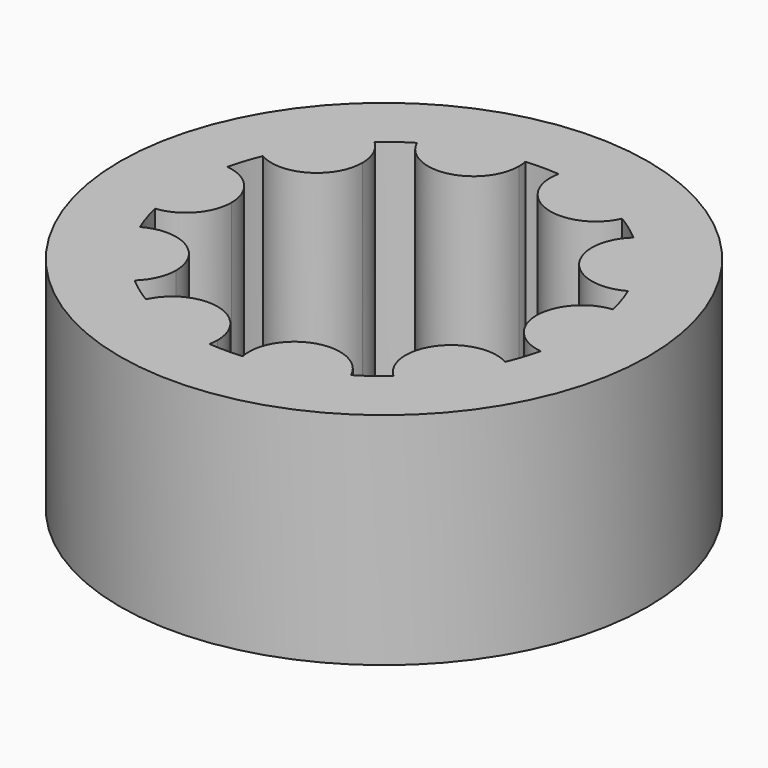
from build123d import *

# Parameters (mm, degrees)
F0_R     = 6
F1_DEPTH = 5


with BuildPart() as f1:
    # F0 (on Top) → F1 (new body)
    with BuildSketch(Plane.XY):
        with Locations((0.1191368553, 0.0803260972)):
            Circle(F0_R)
        with BuildLine():
            ThreePointArc((4.2675466454, 1.8240853161), (4.3988911787, 1.4709025719), (4.5002268275, 1.1079693501))
            ThreePointArc((4.5002268275, 1.1079693501), (5.3073148215, 0.8527258233), (5.6536368553, 0.0803260972))
            ThreePointArc((5.6536368553, 0.0803260972), (5.3073148215, -0.6920736289), (4.5002268275, -0.9473171557))
            ThreePointArc((4.5002268275, -0.9473171557), (4.3988911787, -1.3102503775), (4.2675466454, -1.6634331217))
            ThreePointArc((4.2675466454, -1.6634331217), (4.6528941109, -2.0427704321), (4.79421333, -2.5647075381))
            ThreePointArc((4.79421333, -2.5647075381), (4.1755248273, -3.5119620175), (3.059479548, -3.3261948332))
            ThreePointArc((3.059479548, -3.3261948332), (2.7641704906, -3.5602503775), (2.4503149228, -3.76877884))
            ThreePointArc((2.4503149228, -3.76877884), (2.5204661677, -3.9790445807), (2.54421333, -4.1994282261))
            ThreePointArc((2.54421333, -4.1994282261), (1.6124558319, -5.2288135905), (0.4956212985, -4.4038972987))
            ThreePointArc((0.4956212985, -4.4038972987), (0.1191368553, -4.4196739028), (-0.2573475879, -4.4038972987))
            ThreePointArc((-0.2573475879, -4.4038972987), (-1.5911177, -5.1832961922), (-2.2120412121, -3.76877884))
            ThreePointArc((-2.2120412121, -3.76877884), (-2.52589678, -3.5602503775), (-2.8212058374, -3.3261948332))
            ThreePointArc((-2.8212058374, -3.3261948332), (-4.3583677, -3.1727713816), (-4.0292729348, -1.6634331217))
            ThreePointArc((-4.0292729348, -1.6634331217), (-4.160617468, -1.3102503775), (-4.2619531169, -0.9473171557))
            ThreePointArc((-4.2619531169, -0.9473171557), (-5.4153631447, 0.0803260972), (-4.2619531169, 1.1079693501))
            ThreePointArc((-4.2619531169, 1.1079693501), (-4.160617468, 1.4709025719), (-4.0292729348, 1.8240853161))
            ThreePointArc((-4.0292729348, 1.8240853161), (-4.3583677, 3.333423576), (-2.8212058374, 3.4868470276))
            ThreePointArc((-2.8212058374, 3.4868470276), (-2.52589678, 3.7209025719), (-2.2120412121, 3.9294310345))
            ThreePointArc((-2.2120412121, 3.9294310345), (-1.5911177, 5.3439483866), (-0.2573475879, 4.5645494931))
            ThreePointArc((-0.2573475879, 4.5645494931), (0.1191368553, 4.5803260972), (0.4956212985, 4.5645494931))
            ThreePointArc((0.4956212985, 4.5645494931), (1.6124558319, 5.3894657849), (2.54421333, 4.3600804205))
            ThreePointArc((2.54421333, 4.3600804205), (2.5204661677, 4.1396967751), (2.4503149228, 3.9294310345))
            ThreePointArc((2.4503149228, 3.9294310345), (2.7641704906, 3.7209025719), (3.059479548, 3.4868470276))
            ThreePointArc((3.059479548, 3.4868470276), (4.1755248273, 3.6726142119), (4.79421333, 2.7253597325))
            ThreePointArc((4.79421333, 2.7253597325), (4.6528941109, 2.2034226265), (4.2675466454, 1.8240853161))
        make_face(mode=Mode.SUBTRACT)
        with BuildLine():
            ThreePointArc((4.5002268275, -0.9473171557), (4.5893105027, -0.4369239028), (4.6191368553, 0.0803260972))
            ThreePointArc((4.6191368553, 0.0803260972), (4.5893105027, 0.5975760972), (4.5002268275, 1.1079693501))
            ThreePointArc((4.5002268275, 1.1079693501), (3.5846368553, 0.0803260972), (4.5002268275, -0.9473171557))
        make_face()
        with BuildLine():
            ThreePointArc((4.5002268275, 1.1079693501), (4.5893105027, 0.5975760972), (4.6191368553, 0.0803260972))
            ThreePointArc((4.6191368553, 0.0803260972), (4.5893105027, -0.4369239028), (4.5002268275, -0.9473171557))
            ThreePointArc((4.5002268275, -0.9473171557), (5.3073148215, -0.6920736289), (5.6536368553, 0.0803260972))
            ThreePointArc((5.6536368553, 0.0803260972), (5.3073148215, 0.8527258233), (4.5002268275, 1.1079693501))
        make_face()
        with BuildLine():
            ThreePointArc((3.059479548, 3.4868470276), (2.9227852493, 2.117295889), (4.2675466454, 1.8240853161))
            ThreePointArc((4.2675466454, 1.8240853161), (3.75971333, 2.7253597325), (3.059479548, 3.4868470276))
        make_face()
        with BuildLine():
            ThreePointArc((3.059479548, 3.4868470276), (3.75971333, 2.7253597325), (4.2675466454, 1.8240853161))
            ThreePointArc((4.2675466454, 1.8240853161), (4.6528941109, 2.2034226265), (4.79421333, 2.7253597325))
            ThreePointArc((4.79421333, 2.7253597325), (4.1755248273, 3.6726142119), (3.059479548, 3.4868470276))
        make_face()
        with BuildLine():
            ThreePointArc((4.79421333, -2.5647075381), (4.6528941109, -2.0427704321), (4.2675466454, -1.6634331217))
            ThreePointArc((4.2675466454, -1.6634331217), (3.75971333, -2.5647075381), (3.059479548, -3.3261948332))
            ThreePointArc((3.059479548, -3.3261948332), (4.1755248273, -3.5119620175), (4.79421333, -2.5647075381))
        make_face()
        with BuildLine():
            ThreePointArc((3.059479548, -3.3261948332), (3.75971333, -2.5647075381), (4.2675466454, -1.6634331217))
            ThreePointArc((4.2675466454, -1.6634331217), (2.9227852493, -1.9566436946), (3.059479548, -3.3261948332))
        make_face()
        with BuildLine():
            ThreePointArc((0.4956212985, 4.5645494931), (1.1900352493, 3.3762124544), (2.4503149228, 3.9294310345))
            ThreePointArc((2.4503149228, 3.9294310345), (1.50971333, 4.3600804205), (0.4956212985, 4.5645494931))
        make_face()
        with BuildLine():
            ThreePointArc((0.4956212985, 4.5645494931), (1.50971333, 4.3600804205), (2.4503149228, 3.9294310345))
            ThreePointArc((2.4503149228, 3.9294310345), (2.5204661677, 4.1396967751), (2.54421333, 4.3600804205))
            ThreePointArc((2.54421333, 4.3600804205), (1.6124558319, 5.3894657849), (0.4956212985, 4.5645494931))
        make_face()
        with BuildLine():
            ThreePointArc((2.54421333, -4.1994282261), (2.5204661677, -3.9790445807), (2.4503149228, -3.76877884))
            ThreePointArc((2.4503149228, -3.76877884), (1.50971333, -4.1994282261), (0.4956212985, -4.4038972987))
            ThreePointArc((0.4956212985, -4.4038972987), (1.6124558319, -5.2288135905), (2.54421333, -4.1994282261))
        make_face()
        with BuildLine():
            ThreePointArc((0.4956212985, -4.4038972987), (1.50971333, -4.1994282261), (2.4503149228, -3.76877884))
            ThreePointArc((2.4503149228, -3.76877884), (1.1900352493, -3.21556026), (0.4956212985, -4.4038972987))
        make_face()
        with BuildLine():
            ThreePointArc((-0.2369396194, 4.3600804205), (-0.242054255, 4.4628229225), (-0.2573475879, 4.5645494931))
            ThreePointArc((-0.2573475879, 4.5645494931), (-1.2714396194, 4.3600804205), (-2.2120412121, 3.9294310345))
            ThreePointArc((-2.2120412121, 3.9294310345), (-1.051055974, 3.3493275829), (-0.2369396194, 4.3600804205))
        make_face()
        with BuildLine():
            ThreePointArc((-2.2120412121, 3.9294310345), (-1.2714396194, 4.3600804205), (-0.2573475879, 4.5645494931))
            ThreePointArc((-0.2573475879, 4.5645494931), (-1.5911177, 5.3439483866), (-2.2120412121, 3.9294310345))
        make_face()
        with BuildLine():
            ThreePointArc((-2.2120412121, -3.76877884), (-1.5911177, -5.1832961922), (-0.2573475879, -4.4038972987))
            ThreePointArc((-0.2573475879, -4.4038972987), (-1.2714396194, -4.1994282261), (-2.2120412121, -3.76877884))
        make_face()
        with BuildLine():
            ThreePointArc((-2.2120412121, -3.76877884), (-1.2714396194, -4.1994282261), (-0.2573475879, -4.4038972987))
            ThreePointArc((-0.2573475879, -4.4038972987), (-0.242054255, -4.302170728), (-0.2369396194, -4.1994282261))
            ThreePointArc((-0.2369396194, -4.1994282261), (-1.051055974, -3.1886753885), (-2.2120412121, -3.76877884))
        make_face()
        with BuildLine():
            ThreePointArc((-2.4869396194, 2.7253597325), (-2.57418514, 3.1411712298), (-2.8212058374, 3.4868470276))
            ThreePointArc((-2.8212058374, 3.4868470276), (-3.5214396194, 2.7253597325), (-4.0292729348, 1.8240853161))
            ThreePointArc((-4.0292729348, 1.8240853161), (-2.9995025134, 1.8321789516), (-2.4869396194, 2.7253597325))
        make_face()
        with BuildLine():
            ThreePointArc((-4.0292729348, 1.8240853161), (-3.5214396194, 2.7253597325), (-2.8212058374, 3.4868470276))
            ThreePointArc((-2.8212058374, 3.4868470276), (-4.3583677, 3.333423576), (-4.0292729348, 1.8240853161))
        make_face()
        with BuildLine():
            ThreePointArc((-4.0292729348, -1.6634331217), (-4.3583677, -3.1727713816), (-2.8212058374, -3.3261948332))
            ThreePointArc((-2.8212058374, -3.3261948332), (-3.5214396194, -2.5647075381), (-4.0292729348, -1.6634331217))
        make_face()
        with BuildLine():
            ThreePointArc((-4.0292729348, -1.6634331217), (-3.5214396194, -2.5647075381), (-2.8212058374, -3.3261948332))
            ThreePointArc((-2.8212058374, -3.3261948332), (-2.57418514, -2.9805190354), (-2.4869396194, -2.5647075381))
            ThreePointArc((-2.4869396194, -2.5647075381), (-2.9995025134, -1.6715267572), (-4.0292729348, -1.6634331217))
        make_face()
        with BuildLine():
            ThreePointArc((-3.3463631447, 0.0803260972), (-3.6084634186, 0.7685040634), (-4.2619531169, 1.1079693501))
            ThreePointArc((-4.2619531169, 1.1079693501), (-4.3808631447, 0.0803260972), (-4.2619531169, -0.9473171557))
            ThreePointArc((-4.2619531169, -0.9473171557), (-3.6084634186, -0.607851869), (-3.3463631447, 0.0803260972))
        make_face()
        with BuildLine():
            ThreePointArc((-4.2619531169, -0.9473171557), (-4.3808631447, 0.0803260972), (-4.2619531169, 1.1079693501))
            ThreePointArc((-4.2619531169, 1.1079693501), (-5.4153631447, 0.0803260972), (-4.2619531169, -0.9473171557))
        make_face()
    extrude(amount=F1_DEPTH)


solid = f1.part
